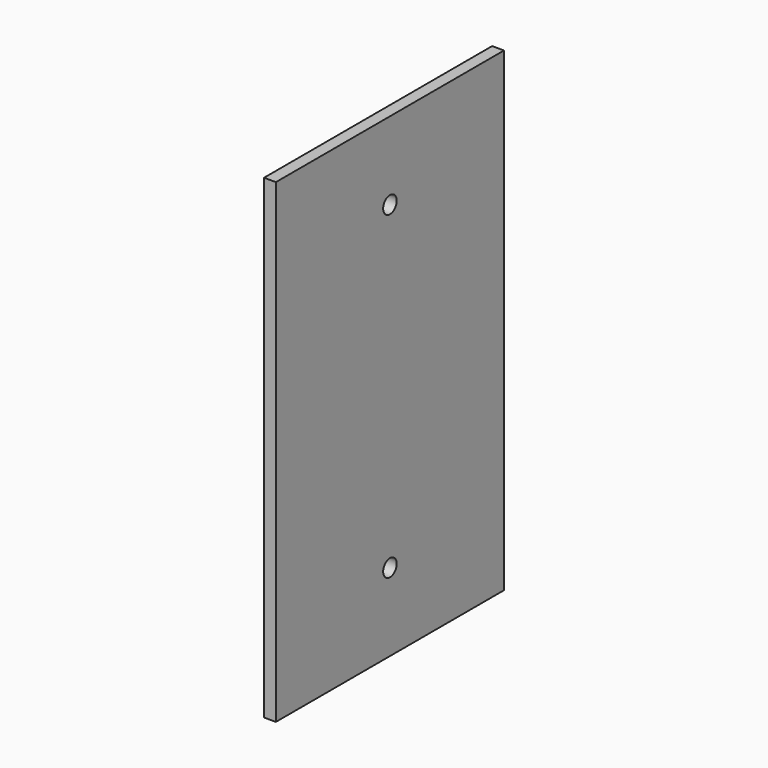
from build123d import *

# Parameters (mm, degrees)
F1_DEPTH = 76.2
F2_R     = 4.5318999151
F3_DEPTH = 6.351


# Not quite as in the source:
# - a feature names something its author has since deleted; it is built from what else it names


with BuildPart() as f1:
    # F0 (on Front) → F1 (new body, symmetric)
    with BuildSketch(Plane.XZ):
        Polygon((0, -127), (0, 0), (0, 127), (-6.35, 127), (-6.35, 0), (-6.35, -127), align=None)
    extrude(amount=F1_DEPTH, both=True)

    # F2 (on face) → F3 (cut, through all)
    with BuildSketch(Plane.YZ):
        with Locations((0, -85.4202)):
            Circle(F2_R)
        with Locations((0, 85.4202)):
            Circle(F2_R)
    extrude(amount=-F3_DEPTH, mode=Mode.SUBTRACT)


solid = f1.part
